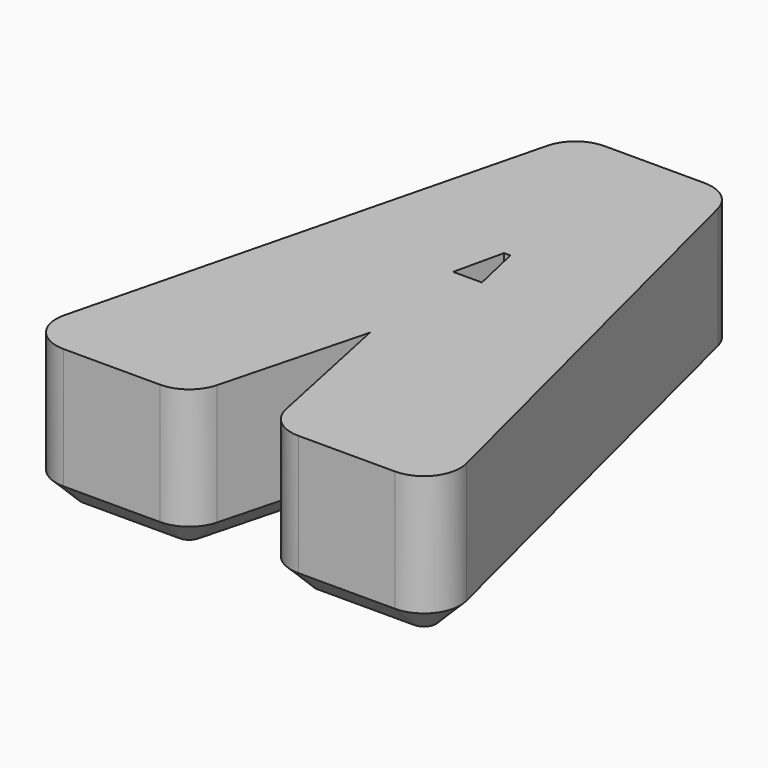
from build123d import *

# Parameters (mm, degrees)
F1_DEPTH     = 30
F3_DEPTH     = 30
F4_DEPTH     = 25
F5_T1_DEPTH  = 97.9548533656
F5_T3_DEPTH  = 20
F5_T5_DEPTH  = 20.7033743208
F5_T7_DEPTH  = 97.9794901198
F5_T9_DEPTH  = 20
F5_T12_ANGLE = 75.8911885194
F5_T14_ANGLE = 104.1088114806
F5_T16_ANGLE = 75.2928746344
F5_T20_DEPTH = 43.6443917162
F5_T23_ANGLE = 75.8339831116
F5_T25_ANGLE = 104.1660168884
F5_T27_ANGLE = 78.1908320725
F5_T31_DEPTH = 42.9024259572
F5_T37_DEPTH = 42.9024259572
F5_T41_DEPTH = 43.6443917162


# Not quite as in the source:
# - a fillet or chamfer that OpenCascade refuses, or shapes differently, is made with other operations: its cross-section is extruded or revolved along the edge and cut away or added
# - the program builds the solid bodies; features that only make, move or delete a surface that nothing else refers to are left out


with BuildPart() as f1:
    # F0 (on Top) → F1 (new body)
    with BuildSketch(Plane.XY):
        with BuildLine():
            Line((9.3227045948, 64.7266464915), (-11.3806697261, 64.7266464915))
            ThreePointArc((-11.3806697261, 64.7266464915), (-15.9925167381, 63.1411090315), (-18.6544287642, 59.0548777281))
            Line((-18.6544287642, 59.0548777281), (-42.5323117917, -35.9451222719))
            ThreePointArc((-42.5323117917, -35.9451222719), (-41.1730152936, -42.3852005206), (-35.2585527536, -45.2733535085))
            Line((-35.2585527536, -45.2733535085), (-15.2585527536, -45.2733535085))
            ThreePointArc((-15.2585527536, -45.2733535085), (-10.6776494918, -43.7118150354), (-8.004281346, -39.6774402567))
            Line((-8.004281346, -39.6774402567), (-0.1883919579, -9.9001294455))
            Line((-0.1883919579, -9.9001294455), (5.9601953638, -39.3082485958))
            ThreePointArc((5.9601953638, -39.3082485958), (8.571852392, -43.5940799733), (13.3014552741, -45.2733535085))
            Line((13.3014552741, -45.2733535085), (33.3014552741, -45.2733535085))
            ThreePointArc((33.3014552741, -45.2733535085), (39.2182193635, -42.3822473792), (40.5733853395, -35.9378608981))
            Line((40.5733853395, -35.9378608981), (16.5946346602, 59.0621391019))
            ThreePointArc((16.5946346602, 59.0621391019), (13.9315984654, 63.1434105808), (9.3227045948, 64.7266464915))
        make_face()
        with BuildLine():
            ThreePointArc((9.3227045948, 59.7266464915), (10.8590025517, 59.1989011879), (11.7466812833, 57.8384773616))
            Line((11.7466812833, 57.8384773616), (35.7254319626, -37.1615226384))
            ThreePointArc((35.7254319626, -37.1615226384), (35.2737099706, -39.3096514654), (33.3014552741, -40.2733535085))
            Line((33.3014552741, -40.2733535085), (13.3014552741, -40.2733535085))
            ThreePointArc((13.3014552741, -40.2733535085), (11.72492098, -39.7135956635), (10.8543686373, -38.2849852043))
            Line((10.8543686373, -38.2849852043), (3.2176150905, -1.7591059289))
            ThreePointArc((3.2176150905, -1.7591059289), (2.3470627478, -0.3304954698), (0.7705284538, 0.2292623753))
            Line((0.7705284538, 0.2292623753), (-0.7705284538, 0.2292623753))
            ThreePointArc((-0.7705284538, 0.2292623753), (-2.2974962077, -0.2912504491), (-3.188618923, -1.6360420419))
            Line((-3.188618923, -1.6360420419), (-12.8404622844, -38.4080490913))
            ThreePointArc((-12.8404622844, -38.4080490913), (-13.7315849996, -39.7528406842), (-15.2585527536, -40.2733535085))
            Line((-15.2585527536, -40.2733535085), (-35.2585527536, -40.2733535085))
            ThreePointArc((-35.2585527536, -40.2733535085), (-37.2300402669, -39.3106358459), (-37.6831390996, -37.1639430963))
            Line((-37.6831390996, -37.1639430963), (-13.8052560721, 57.8360569037))
            ThreePointArc((-13.8052560721, 57.8360569037), (-12.9179520634, 59.1981340048), (-11.3806697261, 59.7266464915))
            Line((-11.3806697261, 59.7266464915), (9.3227045948, 59.7266464915))
        make_face(mode=Mode.SUBTRACT)
    extrude(amount=F1_DEPTH)

    # F0 (on Top) → F3 (join)
    with BuildSketch(Plane.XY):
        with BuildLine():
            Line((35.7254319626, -37.1615226384), (11.7466812833, 57.8384773616))
            ThreePointArc((11.7466812833, 57.8384773616), (10.8590025517, 59.1989011879), (9.3227045948, 59.7266464915))
            Line((9.3227045948, 59.7266464915), (-11.3806697261, 59.7266464915))
            ThreePointArc((-11.3806697261, 59.7266464915), (-12.9179520634, 59.1981340048), (-13.8052560721, 57.8360569037))
            Line((-13.8052560721, 57.8360569037), (-37.6831390996, -37.1639430963))
            ThreePointArc((-37.6831390996, -37.1639430963), (-37.2300402669, -39.3106358459), (-35.2585527536, -40.2733535085))
            Line((-35.2585527536, -40.2733535085), (-15.2585527536, -40.2733535085))
            ThreePointArc((-15.2585527536, -40.2733535085), (-13.7315849996, -39.7528406842), (-12.8404622844, -38.4080490913))
            Line((-12.8404622844, -38.4080490913), (-3.188618923, -1.6360420419))
            ThreePointArc((-3.188618923, -1.6360420419), (-2.2974962077, -0.2912504491), (-0.7705284538, 0.2292623753))
            Line((-0.7705284538, 0.2292623753), (0.7705284538, 0.2292623753))
            ThreePointArc((0.7705284538, 0.2292623753), (2.3470627478, -0.3304954698), (3.2176150905, -1.7591059289))
            Line((3.2176150905, -1.7591059289), (10.8543686373, -38.2849852043))
            ThreePointArc((10.8543686373, -38.2849852043), (11.72492098, -39.7135956635), (13.3014552741, -40.2733535085))
            Line((13.3014552741, -40.2733535085), (33.3014552741, -40.2733535085))
            ThreePointArc((33.3014552741, -40.2733535085), (35.2737099706, -39.3096514654), (35.7254319626, -37.1615226384))
        make_face()
        Polygon((2.9763113208, 15.0989185788), (-2.9763113208, 15.0989185788), (-0.655874512, 25.3615314645), (0.655874512, 25.3615314645), align=None, mode=Mode.SUBTRACT)
    extrude(amount=F3_DEPTH)

    # F0 (on Top) → F4 (cut)
    with BuildSketch(Plane.XY):
        with BuildLine():
            Line((35.7254319626, -37.1615226384), (11.7466812833, 57.8384773616))
            ThreePointArc((11.7466812833, 57.8384773616), (10.8590025517, 59.1989011879), (9.3227045948, 59.7266464915))
            Line((9.3227045948, 59.7266464915), (-11.3806697261, 59.7266464915))
            ThreePointArc((-11.3806697261, 59.7266464915), (-12.9179520634, 59.1981340048), (-13.8052560721, 57.8360569037))
            Line((-13.8052560721, 57.8360569037), (-37.6831390996, -37.1639430963))
            ThreePointArc((-37.6831390996, -37.1639430963), (-37.2300402669, -39.3106358459), (-35.2585527536, -40.2733535085))
            Line((-35.2585527536, -40.2733535085), (-15.2585527536, -40.2733535085))
            ThreePointArc((-15.2585527536, -40.2733535085), (-13.7315849996, -39.7528406842), (-12.8404622844, -38.4080490913))
            Line((-12.8404622844, -38.4080490913), (-3.188618923, -1.6360420419))
            ThreePointArc((-3.188618923, -1.6360420419), (-2.2974962077, -0.2912504491), (-0.7705284538, 0.2292623753))
            Line((-0.7705284538, 0.2292623753), (0.7705284538, 0.2292623753))
            ThreePointArc((0.7705284538, 0.2292623753), (2.3470627478, -0.3304954698), (3.2176150905, -1.7591059289))
            Line((3.2176150905, -1.7591059289), (10.8543686373, -38.2849852043))
            ThreePointArc((10.8543686373, -38.2849852043), (11.72492098, -39.7135956635), (13.3014552741, -40.2733535085))
            Line((13.3014552741, -40.2733535085), (33.3014552741, -40.2733535085))
            ThreePointArc((33.3014552741, -40.2733535085), (35.2737099706, -39.3096514654), (35.7254319626, -37.1615226384))
        make_face()
        Polygon((2.9763113208, 15.0989185788), (-2.9763113208, 15.0989185788), (-0.655874512, 25.3615314645), (0.655874512, 25.3615314645), align=None, mode=Mode.SUBTRACT)
    extrude(amount=F4_DEPTH, mode=Mode.SUBTRACT)

    # F5: chamfer of 5 on 1 edges, made by hand

    # F5_s2 → F5_t1 (cut)
    with BuildSketch(Plane(origin=(12.8527529512, 51.135669312, 0), x_dir=(0, 0, 1), z_dir=(-0.2437641649, -0.9698345384, 0))):
        Polygon((0, 27.4871722621), (5, 32.4871722621), (0, 32.4871722621), align=None)
    extrude(amount=F5_T1_DEPTH, mode=Mode.SUBTRACT)

    # F5_s4 → F5_t3 (cut)
    with BuildSketch(Plane.YZ.offset(-35.2585527536)):
        Polygon((-40.2733535085, 0), (-45.2733535085, 5), (-45.2733535085, 0), align=None)
    extrude(amount=F5_T3_DEPTH, mode=Mode.SUBTRACT)

    # F5_s6 → F5_t5 (cut)
    with BuildSketch(Plane.YZ.offset(-11.3806697261)):
        Polygon((64.7266464915, 5), (59.7266464915, 0), (64.7266464915, 0), align=None)
    extrude(amount=F5_T5_DEPTH, mode=Mode.SUBTRACT)

    # F5_s8 → F5_t7 (cut)
    with BuildSketch(Plane(origin=(10.9578014799, -43.4130682832, 0), x_dir=(0, 0, 1), z_dir=(-0.2447323481, 0.9695906754, 0))):
        Polygon((5, 30.5444190123), (0, 25.5444190123), (0, 30.5444190123), align=None)
    extrude(amount=F5_T7_DEPTH, mode=Mode.SUBTRACT)

    # F5_s10 → F5_t9 (cut)
    with BuildSketch(Plane.YZ.offset(13.3014552741)):
        Polygon((-40.2733535085, 0), (-45.2733535085, 5), (-45.2733535085, 0), align=None)
    extrude(amount=F5_T9_DEPTH, mode=Mode.SUBTRACT)

    # F5_s11 → F5_t12 (revolve, cut)
    with BuildSketch(Plane.YZ.offset(-11.3806697261)):
        Polygon((59.7266464915, 0), (64.7266464915, 5), (64.7266464915, 0), align=None)
    revolve(axis=Axis((-11.3806697261, 57.2266464915, 0), (0, 0, 1)), revolution_arc=F5_T12_ANGLE, mode=Mode.SUBTRACT)

    # F5_s13 → F5_t14 (revolve, cut)
    with BuildSketch(Plane(origin=(-11.0251300763, -43.864330688, 0), x_dir=(0, 0, 1), z_dir=(0.2437641649, 0.9698345384, 0))):
        Polygon((0, -27.4871722621), (5, -32.4871722621), (0, -32.4871722621), align=None)
    revolve(axis=Axis((-35.2585527536, -37.7733535085, 0), (0, 0, 1)), revolution_arc=F5_T14_ANGLE, mode=Mode.SUBTRACT)

    # F5_s15 → F5_t16 (revolve, cut)
    with BuildSketch(Plane.YZ.offset(-15.2585527536)):
        Polygon((-40.2733535085, 0), (-45.2733535085, 5), (-45.2733535085, 0), align=None)
    revolve(axis=Axis((-15.2585527536, -37.7733535085, 0), (0, 0, 1)), revolution_arc=F5_T16_ANGLE, mode=Mode.SUBTRACT)


with BuildPart() as f5_tool18:
    # F5_s19 → F5_t20 (new body)
    with BuildSketch(Plane(origin=(-10.2591099413, -39.0855973263, 0), x_dir=(0, 0, 1), z_dir=(0.2538782331, 0.9672361877, 0))):
        Polygon((0, -2.6687921481), (5, 2.3312078519), (0, 2.3312078519), align=None)
    extrude(amount=F5_T20_DEPTH)

    split(bisect_by=Plane(origin=(-2.1637067448, -0.4523832276, 0), x_dir=(0, 0, 1), z_dir=(-0.9788346547, -0.2046526783, 0)), keep=Keep.TOP)


with BuildPart() as f1_1:
    add(f1.part)

    # F5_t17: cut F5_tool18
    add(f5_tool18.part, mode=Mode.SUBTRACT)

    # F5_s22 → F5_t23 (revolve, cut)
    with BuildSketch(Plane(origin=(-13.0209491994, 51.5869317168, 0), x_dir=(0, 0, 1), z_dir=(0.2447323481, -0.9695906754, 0))):
        Polygon((5, -30.5444190123), (0, -25.5444190123), (0, -30.5444190123), align=None)
    revolve(axis=Axis((9.3227045948, 57.2266464915, 0), (0, 0, 1)), revolution_arc=F5_T23_ANGLE, mode=Mode.SUBTRACT)

    # F5_s24 → F5_t25 (revolve, cut)
    with BuildSketch(Plane.YZ.offset(33.3014552741)):
        Polygon((-40.2733535085, 0), (-45.2733535085, 5), (-45.2733535085, 0), align=None)
    revolve(axis=Axis((33.3014552741, -37.7733535085, 0), (0, 0, 1)), revolution_arc=F5_T25_ANGLE, mode=Mode.SUBTRACT)

    # F5_s26 → F5_t27 (revolve, cut)
    with BuildSketch(Plane(origin=(8.1239021086, -38.8558653682, 0), x_dir=(0, 0, 1), z_dir=(-0.2046526783, 0.9788346547, 0))):
        Polygon((0, 2.7895074164), (5, -2.2104925836), (0, -2.2104925836), align=None)
    revolve(axis=Axis((13.3014552741, -37.7733535085, 0), (0, 0, 1)), revolution_arc=F5_T27_ANGLE, mode=Mode.SUBTRACT)


with BuildPart() as f5_tool29:
    # F5_s30 → F5_t31 (new body)
    with BuildSketch(Plane(origin=(-0.6561942692, 3.1385159299, 0), x_dir=(0, 0, 1), z_dir=(0.2046526783, -0.9788346547, 0))):
        Polygon((0, -2.7895074164), (5, 2.2104925836), (0, 2.2104925836), align=None)
    extrude(amount=F5_T31_DEPTH)

    split(bisect_by=Plane(origin=(2.2548285953, -0.5918429304, 0), x_dir=(0, 0, 1), z_dir=(0.9672361877, -0.2538782331, 0)), keep=Keep.TOP)


with BuildPart() as f1_2:
    add(f1_1.part)

    # F5_t28: cut F5_tool29
    add(f5_tool29.part, mode=Mode.SUBTRACT)


with BuildPart() as f5_tool35:
    # F5_s36 → F5_t37 (new body)
    with BuildSketch(Plane(origin=(-0.6561942692, 3.1385159299, 0), x_dir=(0, 0, 1), z_dir=(0.2046526783, -0.9788346547, 0))):
        Polygon((0, -2.7895074164), (5, 2.2104925836), (0, 2.2104925836), align=None)
    extrude(amount=F5_T37_DEPTH)

    split(bisect_by=Plane(origin=(2.2548285953, -0.5918429304, 0), x_dir=(0, 0, 1), z_dir=(-0.9672361877, 0.2538782331, 0)), keep=Keep.TOP)


with BuildPart() as f5_tool39:
    # F5_s40 → F5_t41 (new body)
    with BuildSketch(Plane(origin=(-10.2591099413, -39.0855973263, 0), x_dir=(0, 0, 1), z_dir=(0.2538782331, 0.9672361877, 0))):
        Polygon((0, -2.6687921481), (5, 2.3312078519), (0, 2.3312078519), align=None)
    extrude(amount=F5_T41_DEPTH)

    split(bisect_by=Plane(origin=(-2.1637067448, -0.4523832276, 0), x_dir=(0, 0, 1), z_dir=(0.9788346547, 0.2046526783, 0)), keep=Keep.TOP)


with BuildPart() as f5_tool35_1:
    add(f5_tool35.part)

    # F5_t43: intersect F5_tool39
    add(f5_tool39.part, mode=Mode.INTERSECT)


with BuildPart() as f1_3:
    add(f1_2.part)

    # F5_t33: cut F5_tool35
    add(f5_tool35_1.part, mode=Mode.SUBTRACT)


solid = f1_3.part
